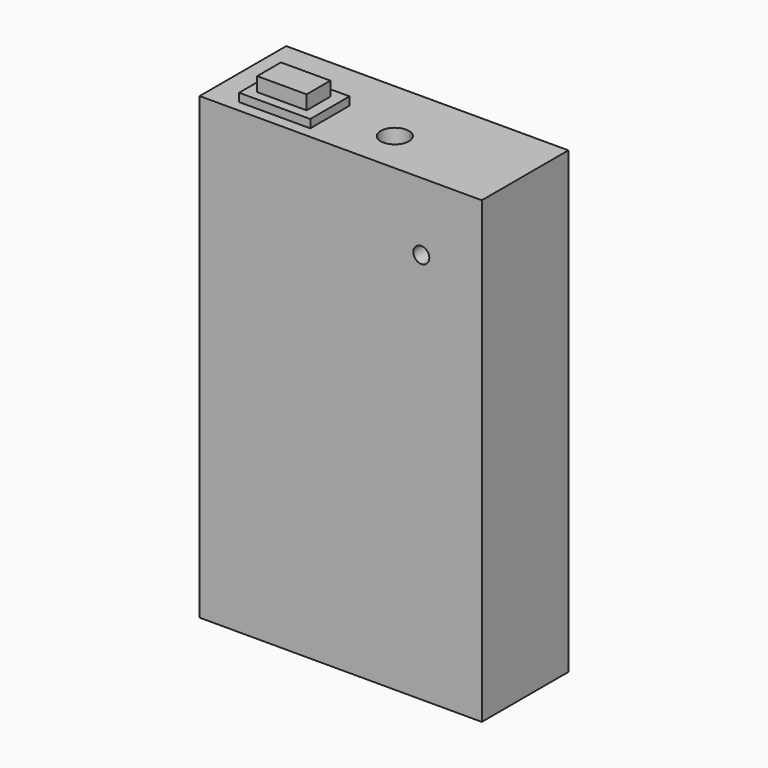
from build123d import *

# Parameters (mm, degrees)
F0_W     = 60
F0_H     = 97.64
F0_R     = 1.7
F1_DEPTH = 23
F3_D     = 6
F3_DEPTH = 8
F3_TIP   = 1.8025818571
F2_W     = 10.5
F2_H     = 6.3
F4_DEPTH = 4.75
F2_W_2   = 15.13
F2_H_2   = 10.44
F5_DEPTH = 1.75


with BuildPart() as f1:
    # F0 (on Front) → F1 (new body)
    with BuildSketch(Plane.XZ):
        with Locations((0.968804583, 14.7747536898)):
            Rectangle(F0_W, F0_H)
        with Locations((18.098804583, 49.1747536898)):
            Circle(F0_R, mode=Mode.SUBTRACT)
    extrude(amount=F1_DEPTH)

    # F3
    with Locations(Plane.XY.offset(63.5947536898)):
        with Locations((5.268804583, -14)):
            Hole(F3_D / 2, depth=F3_DEPTH)
            with Locations((0, 0, -(F3_DEPTH + F3_TIP / 2))):  # 118° drill point
                Cone(0, F3_D / 2, F3_TIP, mode=Mode.SUBTRACT)

    # F2 (on face) → F4 (join)
    with BuildSketch(Plane.XY.offset(63.5947536898)):
        with Locations((-15.0949036926, -15.4)):
            Rectangle(F2_W, F2_H)
    extrude(amount=F4_DEPTH)

    # F2 (on face) → F5 (join)
    with BuildSketch(Plane.XY.offset(63.5947536898)):
        with Locations((-14.9943149662, -15.38)):
            Rectangle(F2_W_2, F2_H_2)
        with Locations((-15.0949036926, -15.4)):
            Rectangle(F2_W, F2_H, mode=Mode.SUBTRACT)
    extrude(amount=F5_DEPTH)


solid = f1.part
